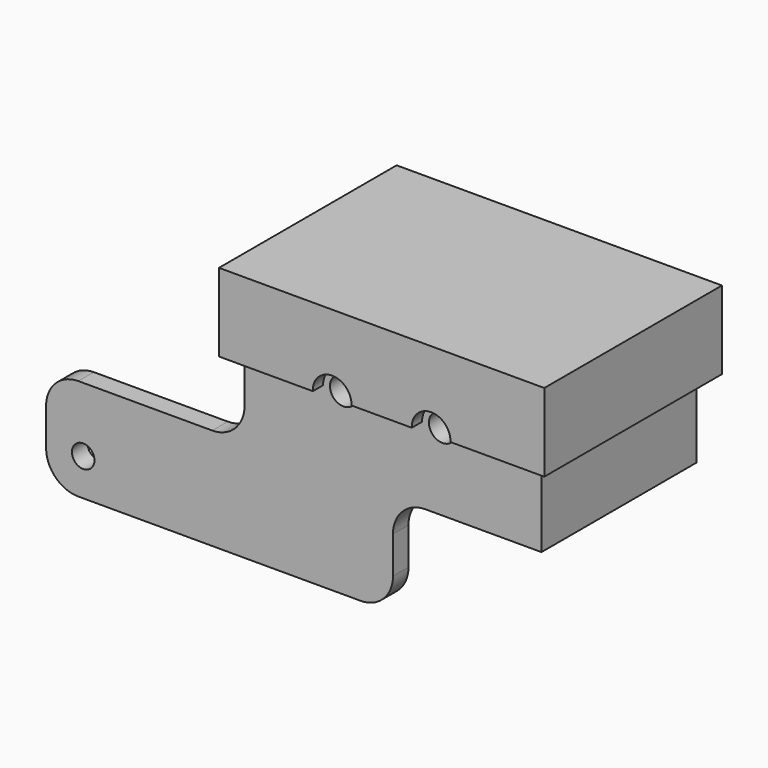
from build123d import *

# Parameters (mm, degrees)
F0_W      = 46
F0_H      = 30
F0_W_2    = 40
F0_H_2    = 20
F1_DEPTH  = 20
F2_R      = 2.1
F3_DEPTH  = 30.001
F4_W      = 2.5
F4_H      = 13.7547671329
F5_DEPTH  = 30.001
F6_W      = 46
F6_H      = 30
F7_DEPTH  = 2
F8_W      = 53.75
F8_H      = 15.75
F8_R      = 1.75
F9_DEPTH  = 3
F10_R     = 5
F11_W     = 50.4
F11_H     = 34.4
F11_W_2   = 46.4
F11_H_2   = 30.4
F11_W_3   = 39
F11_H_3   = 19.5
F12_DEPTH = 2
F13_DEPTH = 1
F14_DEPTH = 10.1
F15_R     = 3
F16_DEPTH = 34.401


with BuildPart() as f1:
    # F0 (on Top) → F1 (new body)
    with BuildSketch(Plane.XY):
        Rectangle(F0_W, F0_H)
        Rectangle(F0_W_2, F0_H_2, mode=Mode.SUBTRACT)
    extrude(amount=F1_DEPTH)

    # F2 (on face) → F3 (cut, through all)
    with BuildSketch(Plane.XZ.offset(15)):
        with Locations((-7.6666666667, 10)):
            Circle(F2_R)
        with Locations((7.6666666667, 10)):
            Circle(F2_R)
    extrude(amount=-F3_DEPTH, mode=Mode.SUBTRACT)

    # F4 (on face) → F5 (cut, through all)
    with BuildSketch(Plane.XZ.offset(15)):
        with Locations((-7.6666666667, 16.8773835665)):
            Rectangle(F4_W, F4_H)
        with Locations((7.6666666667, 16.8773835665)):
            Rectangle(F4_W, F4_H)
    extrude(amount=-F5_DEPTH, mode=Mode.SUBTRACT)

    # F6 (on face) → F7 (join)
    with BuildSketch(Plane(origin=(0, 0, 0), x_dir=(1, 0, 0), z_dir=(0, 0, -1))):
        Rectangle(F6_W, F6_H)
    extrude(amount=F7_DEPTH)

    # F8 (on face) → F9 (join)
    with BuildSketch(Plane.XZ.offset(15)):
        with Locations((-26.875, -9.875)):
            Rectangle(F8_W, F8_H)
        with Locations((-48, -12)):
            Circle(F8_R, mode=Mode.SUBTRACT)
    extrude(amount=-F9_DEPTH)

    # F10
    f10_edges = [f1.edges().sort_by_distance(p)[0] for p in [
        (-53.75, -13.5, -2),
        (-53.75, -13.5, -17.75),
        (-23, -13.5, -2),
        (0, -13.5, -2),
        (0, -13.5, -17.75),
    ]]
    fillet(f10_edges, radius=F10_R)


with BuildPart() as f12:
    # F11 (on face) → F12 (new body)
    with BuildSketch(Plane.XY.offset(20)):
        Rectangle(F11_W, F11_H)
        Rectangle(F11_W_2, F11_H_2, mode=Mode.SUBTRACT)
        Rectangle(F11_W_2, F11_H_2)
        Polygon((-8.9166666667, 15), (-8.9166666667, 10), (-20, 10), (-20, -10), (-8.9166666667, -10), (-8.9166666667, -15), (-23, -15), (-23, 15), align=None, mode=Mode.SUBTRACT)
        Rectangle(F11_W_3, F11_H_3, mode=Mode.SUBTRACT)
        Rectangle(F11_W_3, F11_H_3)
        Polygon((-20, 10), (-8.9166666667, 10), (-8.9166666667, 15), (-23, 15), (-23, -15), (-8.9166666667, -15), (-8.9166666667, -10), (-20, -10), align=None)
    extrude(amount=F12_DEPTH)

    # F11 (on face) → F13 (join)
    with BuildSketch(Plane.XY.offset(20)):
        Rectangle(F11_W_3, F11_H_3)
    extrude(amount=-F13_DEPTH)

    # F11 (on face) → F14 (join)
    with BuildSketch(Plane.XY.offset(20)):
        Rectangle(F11_W, F11_H)
        Rectangle(F11_W_2, F11_H_2, mode=Mode.SUBTRACT)
    extrude(amount=-F14_DEPTH)

    # F15 (on face) → F16 (cut, through all)
    with BuildSketch(Plane.XZ.offset(17.2)):
        with Locations((-7.6666666667, 10)):
            Circle(F15_R)
        with Locations((7.6666666667, 10)):
            Circle(F15_R)
    extrude(amount=-F16_DEPTH, mode=Mode.SUBTRACT)


solid = Compound([f1.part, f12.part])
